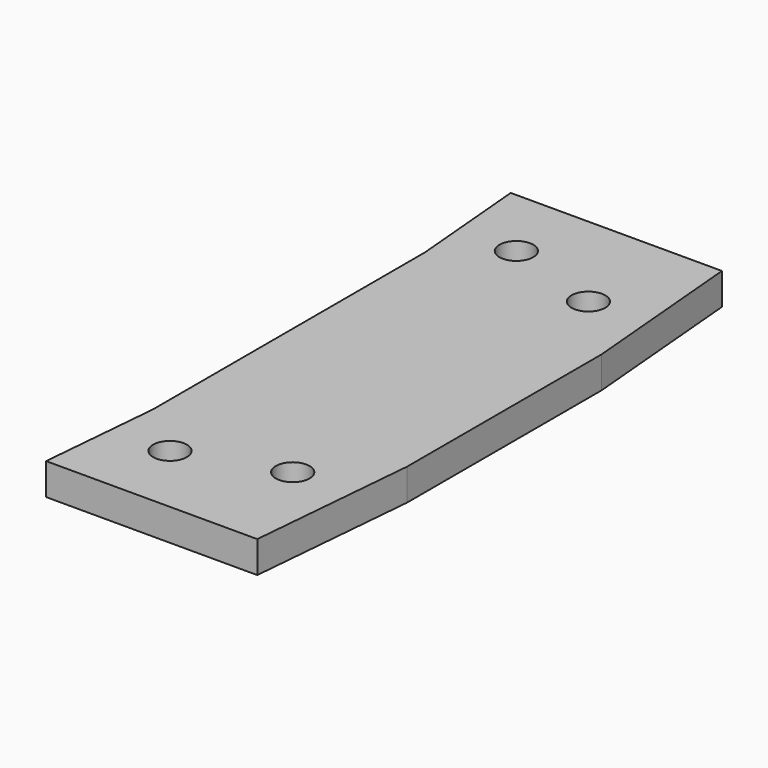
from build123d import *

# Parameters (mm, degrees)
F0_R     = 1.6
F1_DEPTH = 3


# Not quite as in the source:
# - a feature names something its author has since deleted; it is built from what else it names


with BuildPart() as f1:
    # F0 (on Top) → F1 (new body)
    with BuildSketch(Plane.XY):
        Polygon((-3.4388185853, 50.7318324596), (-23.4388185853, 50.7318324596), (-22.4421055113, 39.3393498922), (-22.4421055113, 7.1243150269), (-23.4388185853, -4.2681675404), (-3.4388185853, -4.2681675404), (-2.0389999689, 11.7318324596), (-2.0389999689, 34.7318324596), align=None)
        with Locations((-17.3053888341, 2.7318324596)):
            Circle(F0_R, mode=Mode.SUBTRACT)
        with Locations((-8.0849410565, 5.7318324596)):
            Circle(F0_R, mode=Mode.SUBTRACT)
        with Locations((-17.3053888341, 43.7318324596)):
            Circle(F0_R, mode=Mode.SUBTRACT)
        with Locations((-8.0849410565, 40.7318324596)):
            Circle(F0_R, mode=Mode.SUBTRACT)
    extrude(amount=F1_DEPTH)


solid = f1.part
